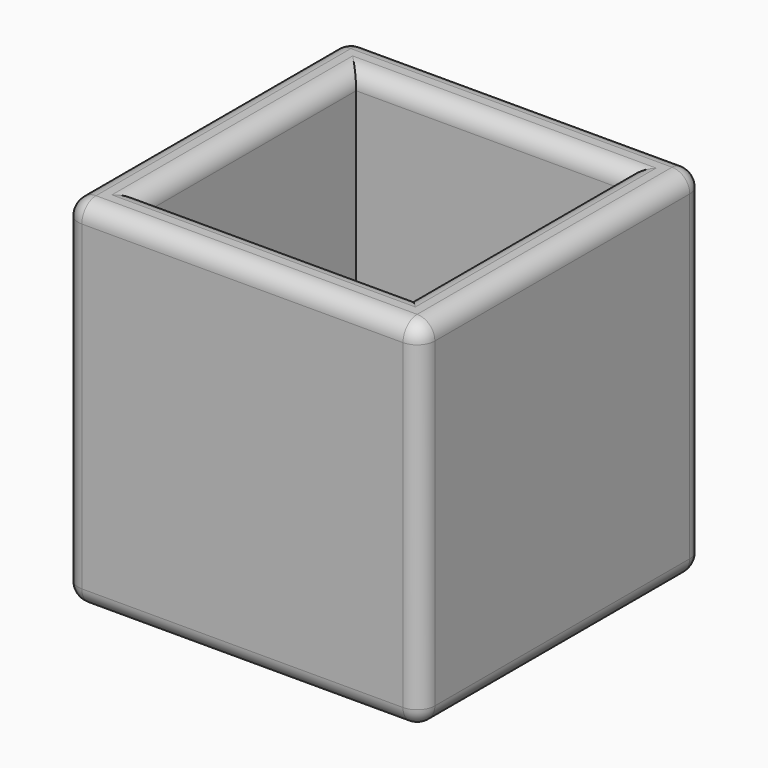
from build123d import *

# Parameters (mm, degrees)
F0_W         = 102.3449450731
F0_H         = 102.3449450731
F1_DEPTH     = 101.6
F2_T         = -12.7
F3_R         = 5.08
F4_T1_DEPTH  = 92.1849450731
F4_T3_DEPTH  = 92.1849450731
F4_T5_DEPTH  = 91.44
F4_S9_W      = 5.08
F4_S9_H      = 5.08
F4_T10_DEPTH = 5.08
F4_S15_W     = 5.08
F4_S15_H     = 5.08
F4_T16_DEPTH = 5.08
F4_S21_W     = 5.08
F4_S21_H     = 5.08
F4_T22_DEPTH = 5.08
F4_S27_W     = 5.08
F4_S27_H     = 5.08
F4_T28_DEPTH = 5.08
F4_T32_ANGLE = 90
F4_T34_ANGLE = 90


# Not quite as in the source:
# - a fillet or chamfer that OpenCascade refuses, or shapes differently, is made with other operations: its cross-section is extruded or revolved along the edge and cut away or added


with BuildPart() as f1:
    # F0 (on Front) → F1 (new body)
    with BuildSketch(Plane.XZ):
        with Locations((-9.3297921121, -3.0156895518)):
            Rectangle(F0_W, F0_H)
    extrude(amount=F1_DEPTH)

    # F2
    f2_openings = [f1.faces().sort_by_distance(p)[0] for p in [
        (-9.329792, -50.8, 48.156783),
    ]]
    offset(amount=F2_T, openings=f2_openings)

    # F3
    f3_edges = [f1.edges().sort_by_distance(p)[0] for p in [
        (41.84268, -50.8, 48.156783),
        (-9.329792, -101.6, 48.156783),
        (41.84268, -101.6, -3.01569),
        (41.84268, -50.8, -54.188162),
        (-9.329792, -101.6, -54.188162),
        (-9.329792, -88.9, 48.156783),
        (-60.502265, -50.8, 48.156783),
        (-9.329792, 0, 48.156783),
        (29.14268, -50.8, 48.156783),
        (-9.329792, -12.7, 48.156783),
        (-47.802265, -50.8, 48.156783),
    ]]
    fillet(f3_edges, radius=F3_R)

    # F4: fillet of radius 5.08 on 3 edges, made by hand

    # F4_s2 → F4_t1 (cut)
    with BuildSketch(Plane.YZ.offset(-55.4222646487)):
        with BuildLine():
            ThreePointArc((-5.08, -54.1881620884), (-1.4878975516, -52.7002645368), (0, -49.1081620884))
            Line((0, -49.1081620884), (0, -54.1881620884))
            Line((0, -54.1881620884), (-5.08, -54.1881620884))
        make_face()
    extrude(amount=F4_T1_DEPTH, mode=Mode.SUBTRACT)

    # F4_s4 → F4_t3 (cut)
    with BuildSketch(Plane.XY.offset(-49.1081620884)):
        with BuildLine():
            ThreePointArc((-60.5022646487, -5.08), (-59.0143670971, -1.4878975516), (-55.4222646487, 0))
            Line((-55.4222646487, 0), (-60.5022646487, 0))
            Line((-60.5022646487, 0), (-60.5022646487, -5.08))
        make_face()
        with BuildLine():
            ThreePointArc((-60.5022646487, -96.52), (-59.0143670971, -100.1121024484), (-55.4222646487, -101.6))
            Line((-55.4222646487, -101.6), (-60.5022646487, -101.6))
            Line((-60.5022646487, -101.6), (-60.5022646487, -96.52))
        make_face()
        with BuildLine():
            ThreePointArc((36.7626804245, 0), (40.3547828729, -1.4878975516), (41.8426804245, -5.08))
            Line((41.8426804245, -5.08), (41.8426804245, 0))
            Line((41.8426804245, 0), (36.7626804245, 0))
        make_face()
    extrude(amount=F4_T3_DEPTH, mode=Mode.SUBTRACT)

    # F4_s6 → F4_t5 (cut)
    with BuildSketch(Plane.XZ.offset(5.08)):
        with BuildLine():
            ThreePointArc((-60.5022646487, -49.1081620884), (-59.0143670971, -52.7002645368), (-55.4222646487, -54.1881620884))
            Line((-55.4222646487, -54.1881620884), (-60.5022646487, -54.1881620884))
            Line((-60.5022646487, -54.1881620884), (-60.5022646487, -49.1081620884))
        make_face()
    extrude(amount=F4_T5_DEPTH, mode=Mode.SUBTRACT)


with BuildPart() as f4_tool8:
    # F4_s9 → F4_t10 (new body)
    with BuildSketch(Plane.YZ.offset(-55.4222646487)):
        with Locations((-99.06, 45.6167829847)):
            Rectangle(F4_S9_W, F4_S9_H)
    extrude(amount=-F4_T10_DEPTH)

    # F4_s11 → F4_t12 (revolve, cut)
    with BuildSketch(Plane(origin=(-55.4222646487, -96.52, 43.0767829847), x_dir=(0, 0.7071067812, -0.7071067812), z_dir=(0, 0.7071067812, 0.7071067812))):
        with BuildLine():
            ThreePointArc((0, -5.08), (5.08, 0), (0, 5.08))
            Line((0, 5.08), (0, -5.08))
        make_face()
    revolve(axis=Axis((-55.4222646487, -96.52, 43.0767829847), (-1, 0, 0)), mode=Mode.SUBTRACT)


with BuildPart() as f1_1:
    add(f1.part)

    # F4_t7: cut F4_tool8
    add(f4_tool8.part, mode=Mode.SUBTRACT)


with BuildPart() as f4_tool14:
    # F4_s15 → F4_t16 (new body)
    with BuildSketch(Plane.YZ.offset(-55.4222646487)):
        with Locations((-2.54, 45.6167829847)):
            Rectangle(F4_S15_W, F4_S15_H)
    extrude(amount=-F4_T16_DEPTH)

    # F4_s17 → F4_t18 (revolve, cut)
    with BuildSketch(Plane(origin=(-55.4222646487, -5.08, 43.0767829847), x_dir=(0, -0.7071067812, -0.7071067812), z_dir=(0, 0.7071067812, -0.7071067812))):
        with BuildLine():
            ThreePointArc((0, -5.08), (5.08, 0), (0, 5.08))
            Line((0, 5.08), (0, -5.08))
        make_face()
    revolve(axis=Axis((-55.4222646487, -5.08, 43.0767829847), (-1, 0, 0)), mode=Mode.SUBTRACT)


with BuildPart() as f1_2:
    add(f1_1.part)

    # F4_t13: cut F4_tool14
    add(f4_tool14.part, mode=Mode.SUBTRACT)


with BuildPart() as f4_tool20:
    # F4_s21 → F4_t22 (new body)
    with BuildSketch(Plane.XZ.offset(5.08)):
        with Locations((39.3026804245, 45.6167829847)):
            Rectangle(F4_S21_W, F4_S21_H)
    extrude(amount=-F4_T22_DEPTH)

    # F4_s23 → F4_t24 (revolve, cut)
    with BuildSketch(Plane(origin=(36.7626804245, -5.08, 43.0767829847), x_dir=(-0.7071067812, 0, -0.7071067812), z_dir=(0.7071067812, 0, -0.7071067812))):
        with BuildLine():
            ThreePointArc((0, -5.08), (5.08, 0), (0, 5.08))
            Line((0, 5.08), (0, -5.08))
        make_face()
    revolve(axis=Axis((36.7626804245, -5.08, 43.0767829847), (0, 1, 0)), mode=Mode.SUBTRACT)


with BuildPart() as f1_3:
    add(f1_2.part)

    # F4_t19: cut F4_tool20
    add(f4_tool20.part, mode=Mode.SUBTRACT)


with BuildPart() as f4_tool26:
    # F4_s27 → F4_t28 (new body)
    with BuildSketch(Plane.YZ.offset(-55.4222646487)):
        with Locations((-2.54, -51.6481620884)):
            Rectangle(F4_S27_W, F4_S27_H)
    extrude(amount=-F4_T28_DEPTH)

    # F4_s29 → F4_t30 (revolve, cut)
    with BuildSketch(Plane(origin=(-55.4222646487, -5.08, -49.1081620884), x_dir=(0, -0.7071067812, 0.7071067812), z_dir=(0, -0.7071067812, -0.7071067812))):
        with BuildLine():
            ThreePointArc((0, -5.08), (5.08, 0), (0, 5.08))
            Line((0, 5.08), (0, -5.08))
        make_face()
    revolve(axis=Axis((-55.4222646487, -5.08, -49.1081620884), (-1, 0, 0)), mode=Mode.SUBTRACT)


with BuildPart() as f1_4:
    add(f1_3.part)

    # F4_t25: cut F4_tool26
    add(f4_tool26.part, mode=Mode.SUBTRACT)

    # F4_s31 → F4_t32 (revolve, cut)
    with BuildSketch(Plane.XZ.offset(96.52)):
        with BuildLine():
            ThreePointArc((-60.5022646487, -49.1081620884), (-59.0143670971, -52.7002645368), (-55.4222646487, -54.1881620884))
            Line((-55.4222646487, -54.1881620884), (-60.5022646487, -54.1881620884))
            Line((-60.5022646487, -54.1881620884), (-60.5022646487, -49.1081620884))
        make_face()
    revolve(axis=Axis((-60.5022646487, -96.52, -49.1081620884), (-1, 0, 0)), revolution_arc=F4_T32_ANGLE, mode=Mode.SUBTRACT)

    # F4_s33 → F4_t34 (revolve, cut)
    with BuildSketch(Plane.YZ.offset(36.7626804245)):
        with BuildLine():
            ThreePointArc((0, -49.1081620884), (-1.4878975516, -52.7002645368), (-5.08, -54.1881620884))
            Line((-5.08, -54.1881620884), (0, -54.1881620884))
            Line((0, -54.1881620884), (0, -49.1081620884))
        make_face()
    revolve(axis=Axis((36.7626804245, 0, -49.1081620884), (0, -1, 0)), revolution_arc=F4_T34_ANGLE, mode=Mode.SUBTRACT)


solid = f1_4.part
